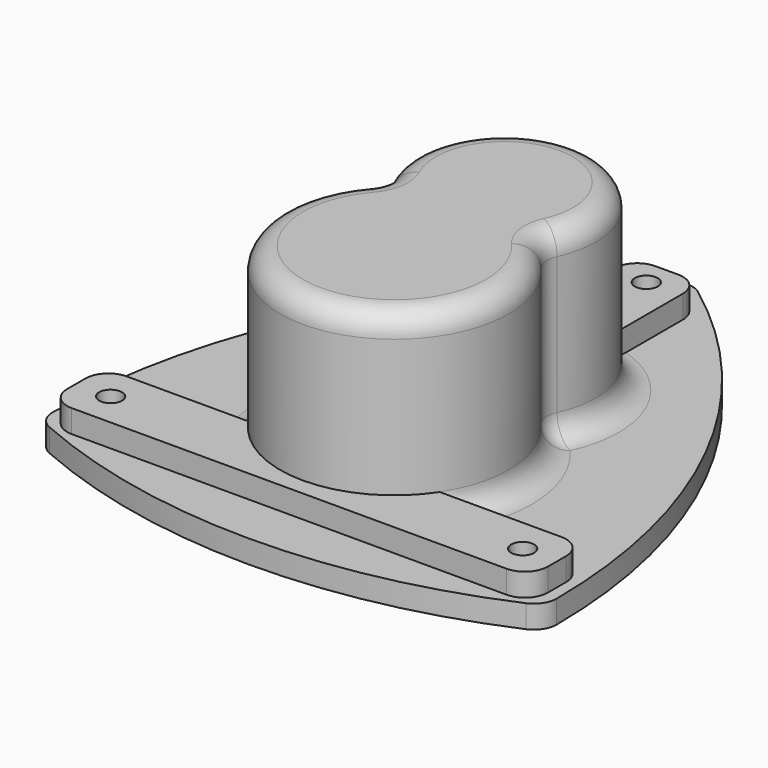
from build123d import *

# Parameters (mm, degrees)
F5_DEPTH  = 5
F3_R      = 20
F2_R      = 25
F2_R_2    = 20
F6_DEPTH  = 50
F7_DEPTH  = 10
F0_R      = 5
F0_R_2    = 2.5
F8_DEPTH  = 5
F9_DEPTH  = 25
F10_R     = 17.5
F11_DEPTH = 40
F12_DEPTH = 5
F13_R     = 5
F14_R     = 5


with BuildPart() as f5:
    # F1 (on Top) → F5 (new body)
    with BuildSketch(Plane.XY):
        with BuildLine():
            ThreePointArc((55.0272203653, -51.5364989145), (41.1164714576, 9.8481618987), (0, 57.5033955377))
            ThreePointArc((0, 57.5033955377), (-41.1164714576, 9.8481618987), (-55.0272203653, -51.5364989145))
            ThreePointArc((-55.0272203653, -51.5364989145), (0, -63.7570226936), (55.0272203653, -51.5364989145))
        make_face()
        with BuildLine():
            ThreePointArc((-45, -45), (-32.3889723065, 4.9444861533), (0, 45))
            ThreePointArc((0, 45), (32.3889723065, 4.9444861533), (45, -45))
            ThreePointArc((45, -45), (0, -53.7570226936), (-45, -45))
        make_face(mode=Mode.SUBTRACT)
        with BuildLine():
            ThreePointArc((45, -45), (32.3889723065, 4.9444861533), (0, 45))
            ThreePointArc((0, 45), (-32.3889723065, 4.9444861533), (-45, -45))
            ThreePointArc((-45, -45), (0, -53.7570226936), (45, -45))
        make_face()
    extrude(amount=F5_DEPTH)

    # F3 (on Top) + F2 (on Top) → F6 (join)
    with BuildSketch(Plane.XY):
        with Locations((0, 6.2429773064)):
            Circle(F3_R)
    with BuildSketch(Plane.XY):
        with Locations((0, -23.7570226936)):
            Circle(F2_R)
        with Locations((0, -23.7570226936)):
            Circle(F2_R_2, mode=Mode.SUBTRACT)
        with Locations((0, -23.7570226936)):
            Circle(F2_R_2)
    extrude(amount=F6_DEPTH)

    # F4 (on Top) → F7 (join)
    with BuildSketch(Plane.XY):
        Polygon((52.5, -37.5), (0, -37.5), (-52.5, -37.5), (-52.5, -52.5), (52.5, -52.5), align=None)
        Polygon((-7.5, 10.6258387864), (0, 10.6258387864), (7.5, 10.6258387864), (7.5, 50.6258387864), (-7.5, 50.6258387864), align=None)
    extrude(amount=F7_DEPTH)

    # F0 (on Top) → F8 (cut)
    with BuildSketch(Plane.XY):
        with Locations((-45, -45)):
            Circle(F0_R)
        with Locations((-45, -45)):
            Circle(F0_R_2, mode=Mode.SUBTRACT)
        with Locations((0, 45)):
            Circle(F0_R)
        with Locations((0, 45)):
            Circle(F0_R_2, mode=Mode.SUBTRACT)
        with Locations((45, -45)):
            Circle(F0_R)
        with Locations((45, -45)):
            Circle(F0_R_2, mode=Mode.SUBTRACT)
    extrude(amount=F8_DEPTH, mode=Mode.SUBTRACT)

    # F0 (on Top) → F9 (cut)
    with BuildSketch(Plane.XY):
        with Locations((-45, -45)):
            Circle(F0_R_2)
        with Locations((0, 45)):
            Circle(F0_R_2)
        with Locations((45, -45)):
            Circle(F0_R_2)
    extrude(amount=F9_DEPTH, mode=Mode.SUBTRACT)

    # F10 (on face) + F2 (on Top) → F11 (cut)
    with BuildSketch(Plane.XY):
        with Locations((0, 6.2429773064)):
            Circle(F10_R)
    with BuildSketch(Plane.XY):
        with Locations((0, -23.7570226936)):
            Circle(F2_R_2)
    extrude(amount=F11_DEPTH, mode=Mode.SUBTRACT)

    # F12 (cut): a face of the model
    f12_faces = [f5.faces().sort_by_distance(p)[0] for p in [
        (0, -12.7665147671, 50),
    ]]
    extrude(f12_faces, amount=-F12_DEPTH, mode=Mode.SUBTRACT)

    # F13
    f13_edges = [f5.edges().sort_by_distance(p)[0] for p in [
        (52.5, -52.5, 7.5),
        (52.5, -37.5, 7.5),
        (55.02722, -51.536499, 2.5),
        (-55.02722, -51.536499, 2.5),
        (-52.5, -52.5, 7.5),
        (-52.5, -37.5, 7.5),
        (-7.5, 50.625839, 7.5),
        (0, 57.503396, 2.5),
        (7.5, 50.625839, 7.5),
    ]]
    fillet(f13_edges, radius=F13_R)

    # F14
    f14_edges = [f5.edges().sort_by_distance(p)[0] for p in [
        (19.138968, 12.04814, 5),
        (-24.779157, -20.441394, 5),
        (24.779157, -20.441394, 5),
        (-19.138968, 12.04814, 5),
        (-16.535946, -5.007023, 25),
        (16.535946, -5.007023, 25),
        (0, 26.242977, 45),
        (0, -48.757023, 45),
    ]]
    fillet(f14_edges, radius=F14_R)


solid = f5.part
